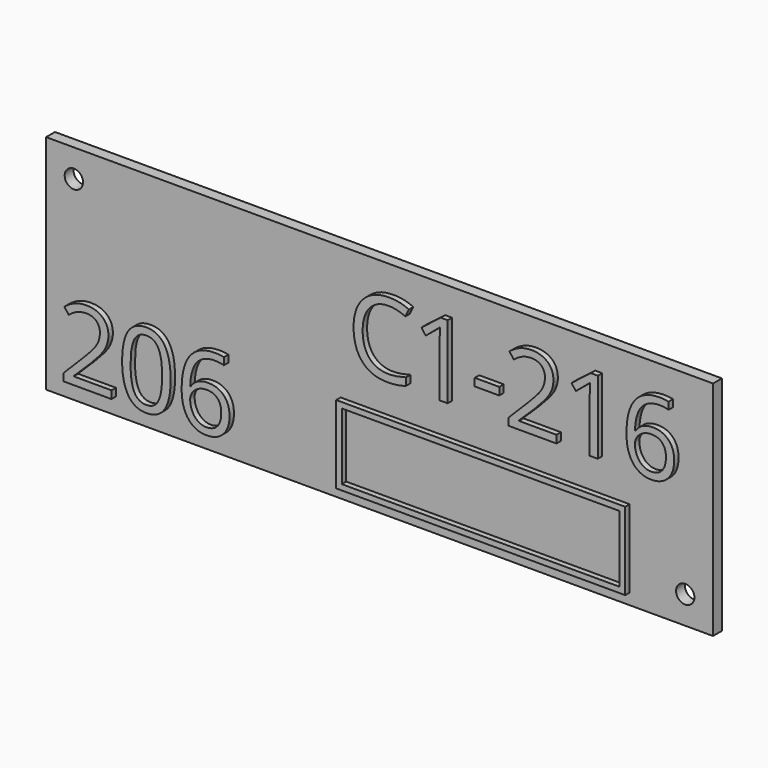
from build123d import *

# Parameters (mm, degrees)
F0_W         = 120
F0_H         = 40
F1_DEPTH     = 2
F3_D         = 3.3
F4_TEXT_SIZE = 18.429641006
F5_DEPTH     = 1
F6_TEXT_SIZE = 18.4837545126
F7_DEPTH     = 1
F8_W         = 52
F8_H         = 14
F8_W_2       = 49.99999962
F8_H_2       = 11.99999962
F9_DEPTH     = 1


# Not quite as in the source:
# - Text() gives the source's letters only with a copy of the font that has no kerning and outlines rounded to 1/6400 em; it was checked with that copy


with BuildPart() as f1:
    # F0 (on Front) → F1 (new body)
    with BuildSketch(Plane.XZ):
        Rectangle(F0_W, F0_H)
    extrude(amount=F1_DEPTH)

    # F3 (through all)
    with Locations(Plane.XZ.offset(2)):
        with Locations((-55, 15), (55, -15)):
            Hole(F3_D / 2)

    # F4 (on face) → F5 (join)
    with BuildSketch(Plane.XZ.offset(2)):
        with Locations((-5, 2)):
            Text('C1-216', F4_TEXT_SIZE, font='Open Sans', text_align=(TextAlign.LEFT, TextAlign.BOTTOM))
    extrude(amount=F5_DEPTH)

    # F6 (on face) → F7 (join)
    with BuildSketch(Plane.XZ.offset(2)):
        with Locations((-57, -17)):
            Text('206', F6_TEXT_SIZE, font='Open Sans', text_align=(TextAlign.LEFT, TextAlign.BOTTOM))
    extrude(amount=F7_DEPTH)

    # F8 (on face) → F9 (join)
    with BuildSketch(Plane.XZ.offset(2)):
        with Locations((19, -11)):
            Rectangle(F8_W, F8_H)
        with Locations((19, -11)):
            Rectangle(F8_W_2, F8_H_2, mode=Mode.SUBTRACT)
    extrude(amount=F9_DEPTH)


solid = f1.part
